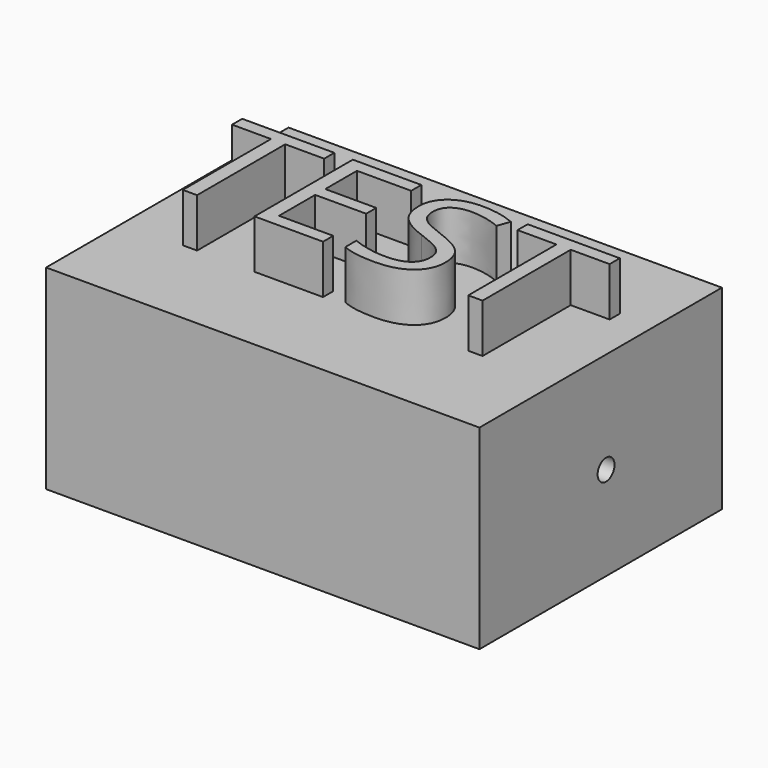
from build123d import *

# Parameters (mm, degrees)
F0_W           = 112.8251589835
F0_H           = 78.903876245
F1_DEPTH       = 50.8
F2_TEXT_SIZE   = 44.8163209043
F3_DEPTH       = 12.7
F5_D           = 5.5
F5_CBORE_D     = 9.75
F5_CBORE_DEPTH = 5


# Not quite as in the source:
# - Text() gives the source's letters only with a copy of the font that has no kerning and outlines rounded to 1/6400 em; it was checked with that copy


with BuildPart() as f1:
    # F0 (on Top) → F1 (new body)
    with BuildSketch(Plane.XY):
        with Locations((5.991531536, -1.751370728)):
            Rectangle(F0_W, F0_H)
    extrude(amount=F1_DEPTH)

    # F2 (on face) → F3 (join)
    with BuildSketch(Plane.XY.offset(50.8)):
        with Locations((-45.3410479558, -16.2156131472)):
            Text('TEST', F2_TEXT_SIZE, font='Open Sans', text_align=(TextAlign.LEFT, TextAlign.BOTTOM))
    extrude(amount=F3_DEPTH)

    # F5 (through all)
    with Locations(Plane(origin=(-50.4210479558, 0, 0), x_dir=(0, -1, 0), z_dir=(-1, 0, 0))):
        with Locations((0, 24.4100000709)):
            CounterBoreHole(F5_D / 2, F5_CBORE_D / 2, F5_CBORE_DEPTH)


solid = f1.part
